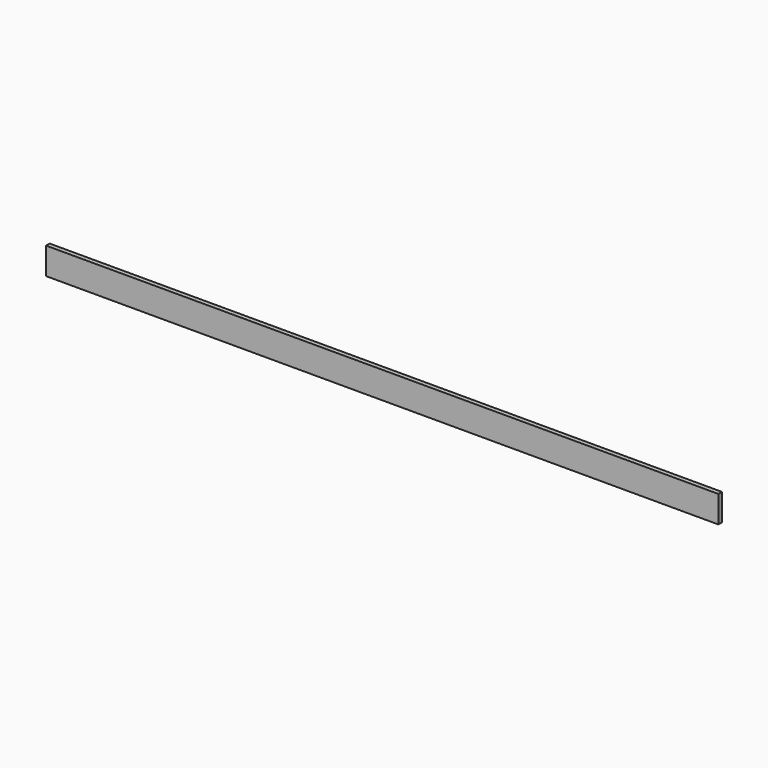
from build123d import *

# Parameters (mm, degrees)
F0_W     = 2
F0_H     = 12
F1_DEPTH = 150


# Not quite as in the source:
# - the program builds the solid bodies; features that only make, move or delete a surface that nothing else refers to are left out


with BuildPart() as f1:
    # F0 (on Right) → F1 (new body, symmetric)
    with BuildSketch(Plane.YZ):
        Rectangle(F0_W, F0_H)
    extrude(amount=F1_DEPTH, both=True)


solid = f1.part
